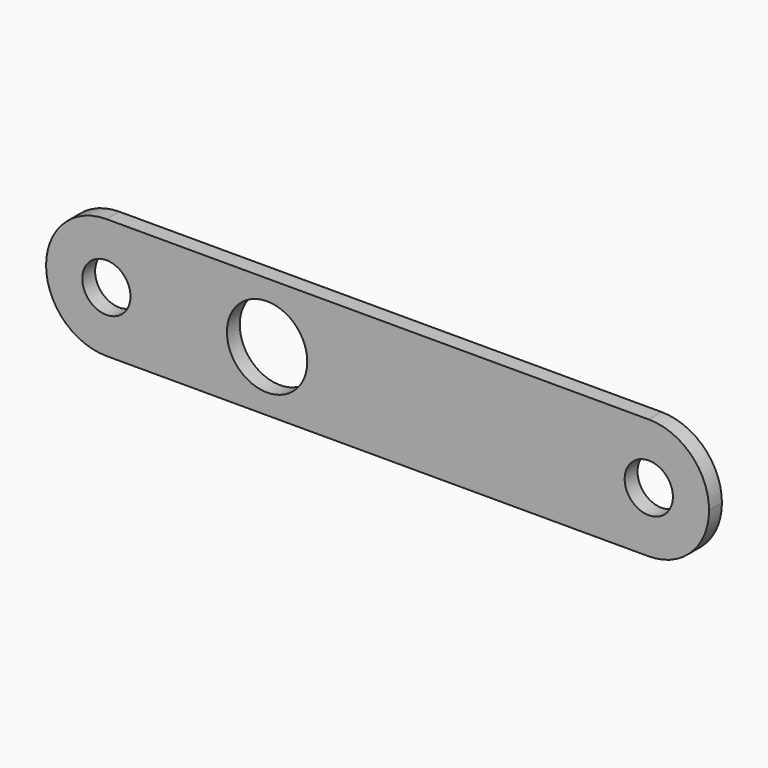
from build123d import *

# Parameters (mm, degrees)
F0_W     = 82.5
F0_H     = 15
F0_R     = 3
F1_DEPTH = 1
F2_R     = 7.49999
F3_R     = 5
F4_DEPTH = 12.5


# Not quite as in the source:
# - a fillet or chamfer is up to 0.001 mm smaller than in the source, because OpenCascade refuses the exact size


with BuildPart() as f1:
    # F0 (on Front) → F1 (new body, symmetric)
    with BuildSketch(Plane.XZ):
        with Locations((33.75, 0)):
            Rectangle(F0_W, F0_H)
        Circle(F0_R, mode=Mode.SUBTRACT)
        with Locations((67.5, 0)):
            Circle(F0_R, mode=Mode.SUBTRACT)
    extrude(amount=F1_DEPTH, both=True)

    # F2 (radius 7.5 in the source; OpenCascade refuses exactly that, so slightly less here)
    f2_edges = [f1.edges().sort_by_distance(p)[0] for p in [
        (75, 0, 7.5),
        (75, 0, -7.5),
        (-7.5, 0, 7.5),
        (-7.5, 0, -7.5),
    ]]
    fillet(f2_edges, radius=F2_R)

    # F3 (on Front) → F4 (cut, symmetric)
    with BuildSketch(Plane.XZ):
        with Locations((20, 0)):
            Circle(F3_R)
    extrude(amount=F4_DEPTH, both=True, mode=Mode.SUBTRACT)


solid = f1.part
